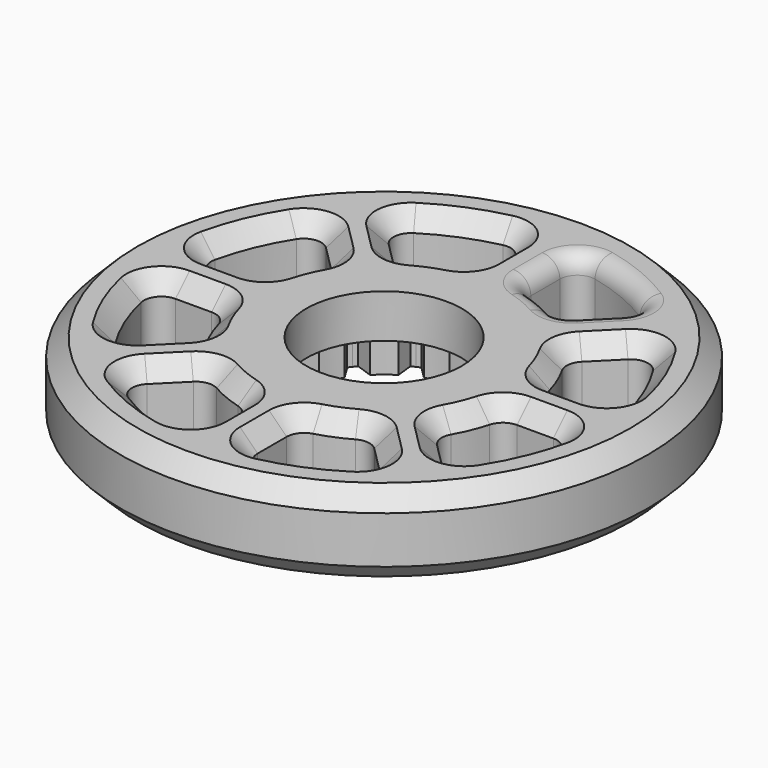
from build123d import *

# Parameters (mm, degrees)
F0_R     = 75
F0_R_2   = 22.1
F1_DEPTH = 23.4
F2_R     = 22.1
F3_DEPTH = 11
F5_DEPTH = 25
F6_F1_R  = 5
F6_F2_R  = 5
F7_SIZE  = 5


with BuildPart() as f1:
    # F0 (on Top) → F1 (new body)
    with BuildSketch(Plane.XY):
        Circle(F0_R)
        Circle(F0_R_2, mode=Mode.SUBTRACT)
    extrude(amount=F1_DEPTH)

    # F2 (on face) → F3 (cut)
    with BuildSketch(Plane(origin=(0, 0, 0), x_dir=(1, 0, 0), z_dir=(0, 0, -1))):
        with BuildLine():
            Line((1.25, -31.4751886412), (2.9, -26.8438074796))
            ThreePointArc((2.9, -26.8438074796), (6.0080652168, -26.3230536289), (9.0342818445, -25.4436976785))
            Line((9.0342818445, -25.4436976785), (12.5303614522, -28.900519751))
            Line((12.5303614522, -28.900519751), (13.6673377822, -28.3805193389))
            Line((13.6673377822, -28.3805193389), (14.782783622, -27.8158104032))
            Line((14.782783622, -27.8158104032), (14.2599012783, -22.9271719916))
            ThreePointArc((14.2599012783, -22.9271719916), (16.8342246502, -21.1094500266), (19.1792133714, -19.0041515057))
            Line((19.1792133714, -19.0041515057), (23.828931144, -20.6017484825))
            Line((23.828931144, -20.6017484825), (24.6276916977, -19.6399287586))
            Line((24.6276916977, -19.6399287586), (25.3876556486, -18.6471697763))
            Line((25.3876556486, -18.6471697763), (22.7954542222, -14.4695289074))
            ThreePointArc((22.7954542222, -14.4695289074), (24.3261594334, -11.7148609562), (25.5254664726, -8.8006000566))
            Line((25.5254664726, -8.8006000566), (30.4078887801, -8.2225482631))
            Line((30.4078887801, -8.2225482631), (30.7102292337, -7.0094094196))
            Line((30.7102292337, -7.0094094196), (30.964191115, -5.7852284827))
            Line((30.964191115, -5.7852284827), (26.8160878895, -3.146018166))
            ThreePointArc((26.8160878895, -3.146018166), (27, 0), (26.8160878895, 3.146018166))
            Line((26.8160878895, 3.146018166), (30.964191115, 5.7852284827))
            Line((30.964191115, 5.7852284827), (30.7102292337, 7.0094094196))
            Line((30.7102292337, 7.0094094196), (30.4078887801, 8.2225482631))
            Line((30.4078887801, 8.2225482631), (25.5254664726, 8.8006000566))
            ThreePointArc((25.5254664726, 8.8006000566), (24.3261594334, 11.7148609562), (22.7954542222, 14.4695289074))
            Line((22.7954542222, 14.4695289074), (25.3876556486, 18.6471697763))
            Line((25.3876556486, 18.6471697763), (24.6276916977, 19.6399287586))
            Line((24.6276916977, 19.6399287586), (23.828931144, 20.6017484825))
            Line((23.828931144, 20.6017484825), (19.1792133714, 19.0041515057))
            ThreePointArc((19.1792133714, 19.0041515057), (16.8342246502, 21.1094500266), (14.2599012783, 22.9271719916))
            Line((14.2599012783, 22.9271719916), (14.782783622, 27.8158104032))
            Line((14.782783622, 27.8158104032), (13.6673377822, 28.3805193389))
            Line((13.6673377822, 28.3805193389), (12.5303614522, 28.900519751))
            Line((12.5303614522, 28.900519751), (9.0342818445, 25.4436976785))
            ThreePointArc((9.0342818445, 25.4436976785), (6.0080652168, 26.3230536289), (2.9, 26.8438074796))
            Line((2.9, 26.8438074796), (1.25, 31.4751886412))
            Line((1.25, 31.4751886412), (0, 31.5))
            Line((0, 31.5), (-1.25, 31.4751886412))
            Line((-1.25, 31.4751886412), (-2.9, 26.8438074796))
            ThreePointArc((-2.9, 26.8438074796), (-6.0080652168, 26.3230536289), (-9.0342818445, 25.4436976785))
            Line((-9.0342818445, 25.4436976785), (-12.5303614522, 28.900519751))
            Line((-12.5303614522, 28.900519751), (-13.6673377822, 28.3805193389))
            Line((-13.6673377822, 28.3805193389), (-14.782783622, 27.8158104032))
            Line((-14.782783622, 27.8158104032), (-14.2599012783, 22.9271719916))
            ThreePointArc((-14.2599012783, 22.9271719916), (-16.8342246502, 21.1094500266), (-19.1792133714, 19.0041515057))
            Line((-19.1792133714, 19.0041515057), (-23.828931144, 20.6017484825))
            Line((-23.828931144, 20.6017484825), (-24.6276916977, 19.6399287586))
            Line((-24.6276916977, 19.6399287586), (-25.3876556486, 18.6471697763))
            Line((-25.3876556486, 18.6471697763), (-22.7954542222, 14.4695289074))
            ThreePointArc((-22.7954542222, 14.4695289074), (-24.3261594334, 11.7148609562), (-25.5254664726, 8.8006000566))
            Line((-25.5254664726, 8.8006000566), (-30.4078887801, 8.2225482631))
            Line((-30.4078887801, 8.2225482631), (-30.7102292337, 7.0094094196))
            Line((-30.7102292337, 7.0094094196), (-30.964191115, 5.7852284827))
            Line((-30.964191115, 5.7852284827), (-26.8160878895, 3.146018166))
            ThreePointArc((-26.8160878895, 3.146018166), (-27, 0), (-26.8160878895, -3.146018166))
            Line((-26.8160878895, -3.146018166), (-30.964191115, -5.7852284827))
            Line((-30.964191115, -5.7852284827), (-30.7102292337, -7.0094094196))
            Line((-30.7102292337, -7.0094094196), (-30.4078887801, -8.2225482631))
            Line((-30.4078887801, -8.2225482631), (-25.5254664726, -8.8006000566))
            ThreePointArc((-25.5254664726, -8.8006000566), (-24.3261594334, -11.7148609562), (-22.7954542222, -14.4695289074))
            Line((-22.7954542222, -14.4695289074), (-25.3876556486, -18.6471697763))
            Line((-25.3876556486, -18.6471697763), (-24.6276916977, -19.6399287586))
            Line((-24.6276916977, -19.6399287586), (-23.828931144, -20.6017484825))
            Line((-23.828931144, -20.6017484825), (-19.1792133714, -19.0041515057))
            ThreePointArc((-19.1792133714, -19.0041515057), (-16.8342246502, -21.1094500266), (-14.2599012783, -22.9271719916))
            Line((-14.2599012783, -22.9271719916), (-14.782783622, -27.8158104032))
            Line((-14.782783622, -27.8158104032), (-13.6673377822, -28.3805193389))
            Line((-13.6673377822, -28.3805193389), (-12.5303614522, -28.900519751))
            Line((-12.5303614522, -28.900519751), (-9.0342818445, -25.4436976785))
            ThreePointArc((-9.0342818445, -25.4436976785), (-6.0080652168, -26.3230536289), (-2.9, -26.8438074796))
            Line((-2.9, -26.8438074796), (-1.25, -31.4751886412))
            Line((-1.25, -31.4751886412), (0, -31.5))
            Line((0, -31.5), (1.25, -31.4751886412))
        make_face()
        Circle(F2_R, mode=Mode.SUBTRACT)
        with BuildLine():
            ThreePointArc((0, -31.5), (0.6251231086, -31.4937965495), (1.25, -31.4751886412))
            Line((1.25, -31.4751886412), (0, -31.5))
        make_face()
        with BuildLine():
            Line((13.6673377822, -28.3805193389), (12.5303614522, -28.900519751))
            ThreePointArc((12.5303614522, -28.900519751), (13.1014297465, -28.6461609749), (13.6673377822, -28.3805193389))
        make_face()
        with BuildLine():
            Line((14.782783622, -27.8158104032), (13.6673377822, -28.3805193389))
            ThreePointArc((13.6673377822, -28.3805193389), (14.2278626653, -28.1036994714), (14.782783622, -27.8158104032))
        make_face()
        with BuildLine():
            ThreePointArc((-13.6673377822, -28.3805193389), (-13.1014297465, -28.6461609749), (-12.5303614522, -28.900519751))
            Line((-12.5303614522, -28.900519751), (-13.6673377822, -28.3805193389))
        make_face()
        with BuildLine():
            Line((24.6276916977, -19.6399287586), (23.828931144, -20.6017484825))
            ThreePointArc((23.828931144, -20.6017484825), (24.2330837617, -20.1248018971), (24.6276916977, -19.6399287586))
        make_face()
        with BuildLine():
            ThreePointArc((-14.782783622, -27.8158104032), (-14.2278626653, -28.1036994714), (-13.6673377822, -28.3805193389))
            Line((-13.6673377822, -28.3805193389), (-14.782783622, -27.8158104032))
        make_face()
        with BuildLine():
            Line((25.3876556486, -18.6471697763), (24.6276916977, -19.6399287586))
            ThreePointArc((24.6276916977, -19.6399287586), (25.0125995279, -19.1473200437), (25.3876556486, -18.6471697763))
        make_face()
        with BuildLine():
            Line((30.7102292337, -7.0094094196), (30.4078887801, -8.2225482631))
            ThreePointArc((30.4078887801, -8.2225482631), (30.5650783387, -7.6174789891), (30.7102292337, -7.0094094196))
        make_face()
        with BuildLine():
            ThreePointArc((-25.3876556486, -18.6471697763), (-25.0125995279, -19.1473200437), (-24.6276916977, -19.6399287586))
            Line((-24.6276916977, -19.6399287586), (-25.3876556486, -18.6471697763))
        make_face()
        with BuildLine():
            Line((30.964191115, -5.7852284827), (30.7102292337, -7.0094094196))
            ThreePointArc((30.7102292337, -7.0094094196), (30.8432842946, -6.3985790549), (30.964191115, -5.7852284827))
        make_face()
        with BuildLine():
            Line((30.7102292337, 7.0094094196), (30.964191115, 5.7852284827))
            ThreePointArc((30.964191115, 5.7852284827), (30.8432842946, 6.3985790549), (30.7102292337, 7.0094094196))
        make_face()
        with BuildLine():
            ThreePointArc((-30.964191115, -5.7852284827), (-30.8432842946, -6.3985790549), (-30.7102292337, -7.0094094196))
            Line((-30.7102292337, -7.0094094196), (-30.964191115, -5.7852284827))
        make_face()
        with BuildLine():
            Line((30.4078887801, 8.2225482631), (30.7102292337, 7.0094094196))
            ThreePointArc((30.7102292337, 7.0094094196), (30.5650783387, 7.6174789891), (30.4078887801, 8.2225482631))
        make_face()
        with BuildLine():
            ThreePointArc((-30.7102292337, 7.0094094196), (-30.8432842946, 6.3985790549), (-30.964191115, 5.7852284827))
            Line((-30.964191115, 5.7852284827), (-30.7102292337, 7.0094094196))
        make_face()
        with BuildLine():
            Line((24.6276916977, 19.6399287586), (25.3876556486, 18.6471697763))
            ThreePointArc((25.3876556486, 18.6471697763), (25.0125995279, 19.1473200437), (24.6276916977, 19.6399287586))
        make_face()
        with BuildLine():
            ThreePointArc((-30.4078887801, 8.2225482631), (-30.5650783387, 7.6174789891), (-30.7102292337, 7.0094094196))
            Line((-30.7102292337, 7.0094094196), (-30.4078887801, 8.2225482631))
        make_face()
        with BuildLine():
            Line((23.828931144, 20.6017484825), (24.6276916977, 19.6399287586))
            ThreePointArc((24.6276916977, 19.6399287586), (24.2330837617, 20.1248018971), (23.828931144, 20.6017484825))
        make_face()
        with BuildLine():
            ThreePointArc((-24.6276916977, 19.6399287586), (-25.0125995279, 19.1473200437), (-25.3876556486, 18.6471697763))
            Line((-25.3876556486, 18.6471697763), (-24.6276916977, 19.6399287586))
        make_face()
        with BuildLine():
            Line((13.6673377822, 28.3805193389), (14.782783622, 27.8158104032))
            ThreePointArc((14.782783622, 27.8158104032), (14.2278626653, 28.1036994714), (13.6673377822, 28.3805193389))
        make_face()
        with BuildLine():
            ThreePointArc((-23.828931144, 20.6017484825), (-24.2330837617, 20.1248018971), (-24.6276916977, 19.6399287586))
            Line((-24.6276916977, 19.6399287586), (-23.828931144, 20.6017484825))
        make_face()
        with BuildLine():
            Line((12.5303614522, 28.900519751), (13.6673377822, 28.3805193389))
            ThreePointArc((13.6673377822, 28.3805193389), (13.1014297465, 28.6461609749), (12.5303614522, 28.900519751))
        make_face()
        with BuildLine():
            ThreePointArc((-13.6673377822, 28.3805193389), (-14.2278626653, 28.1036994714), (-14.782783622, 27.8158104032))
            Line((-14.782783622, 27.8158104032), (-13.6673377822, 28.3805193389))
        make_face()
        with BuildLine():
            Line((0, 31.5), (1.25, 31.4751886412))
            ThreePointArc((1.25, 31.4751886412), (0.6251231086, 31.4937965495), (0, 31.5))
        make_face()
        with BuildLine():
            ThreePointArc((-12.5303614522, 28.900519751), (-13.1014297465, 28.6461609749), (-13.6673377822, 28.3805193389))
            Line((-13.6673377822, 28.3805193389), (-12.5303614522, 28.900519751))
        make_face()
        with BuildLine():
            Line((-1.25, 31.4751886412), (0, 31.5))
            ThreePointArc((0, 31.5), (-0.6251231086, 31.4937965495), (-1.25, 31.4751886412))
        make_face()
    extrude(amount=-F3_DEPTH, mode=Mode.SUBTRACT)

    # F4 (on face) → F5 (cut)
    with BuildSketch(Plane(origin=(0, 0, 0), x_dir=(1, 0, 0), z_dir=(0, 0, -1))):
        with BuildLine():
            ThreePointArc((-39.3817561055, 7.0055182569), (-36.9551813005, 15.3073372946), (-32.8007562624, 22.893457332))
            Line((-32.8007562624, 22.893457332), (-47.0898732753, 37.1825743449))
            ThreePointArc((-47.0898732753, 37.1825743449), (-55.4327719507, 22.9610059419), (-59.5896191795, 7.0055182569))
            Line((-59.5896191795, 7.0055182569), (-39.3817561055, 7.0055182569))
        make_face()
        with BuildLine():
            Line((-7.0055182569, 39.3817561055), (-7.0055182569, 59.5896191795))
            ThreePointArc((-7.0055182569, 59.5896191795), (-22.9610059419, 55.4327719507), (-37.1825743449, 47.0898732753))
            Line((-37.1825743449, 47.0898732753), (-22.893457332, 32.8007562624))
            ThreePointArc((-22.893457332, 32.8007562624), (-15.3073372946, 36.9551813005), (-7.0055182569, 39.3817561055))
        make_face()
        with BuildLine():
            ThreePointArc((37.1825743449, 47.0898732753), (22.9610059419, 55.4327719507), (7.0055182569, 59.5896191795))
            Line((7.0055182569, 59.5896191795), (7.0055182569, 39.3817561055))
            ThreePointArc((7.0055182569, 39.3817561055), (15.3073372946, 36.9551813005), (22.893457332, 32.8007562624))
            Line((22.893457332, 32.8007562624), (37.1825743449, 47.0898732753))
        make_face()
        with BuildLine():
            Line((39.3817561055, 7.0055182569), (59.5896191795, 7.0055182569))
            ThreePointArc((59.5896191795, 7.0055182569), (55.4327719507, 22.9610059419), (47.0898732753, 37.1825743449))
            Line((47.0898732753, 37.1825743449), (32.8007562624, 22.893457332))
            ThreePointArc((32.8007562624, 22.893457332), (36.9551813005, 15.3073372946), (39.3817561055, 7.0055182569))
        make_face()
        with BuildLine():
            Line((32.8007562624, -22.893457332), (47.0898732753, -37.1825743449))
            ThreePointArc((47.0898732753, -37.1825743449), (55.4327719507, -22.9610059419), (59.5896191795, -7.0055182569))
            Line((59.5896191795, -7.0055182569), (39.3817561055, -7.0055182569))
            ThreePointArc((39.3817561055, -7.0055182569), (36.9551813005, -15.3073372946), (32.8007562624, -22.893457332))
        make_face()
        with BuildLine():
            Line((7.0055182569, -39.3817561055), (7.0055182569, -59.5896191795))
            ThreePointArc((7.0055182569, -59.5896191795), (22.9610059419, -55.4327719507), (37.1825743449, -47.0898732753))
            Line((37.1825743449, -47.0898732753), (22.893457332, -32.8007562624))
            ThreePointArc((22.893457332, -32.8007562624), (15.3073372946, -36.9551813005), (7.0055182569, -39.3817561055))
        make_face()
        with BuildLine():
            Line((-22.893457332, -32.8007562624), (-37.1825743449, -47.0898732753))
            ThreePointArc((-37.1825743449, -47.0898732753), (-22.9610059419, -55.4327719507), (-7.0055182569, -59.5896191795))
            Line((-7.0055182569, -59.5896191795), (-7.0055182569, -39.3817561055))
            ThreePointArc((-7.0055182569, -39.3817561055), (-15.3073372946, -36.9551813005), (-22.893457332, -32.8007562624))
        make_face()
        with BuildLine():
            Line((-39.3817561055, -7.0055182569), (-59.5896191795, -7.0055182569))
            ThreePointArc((-59.5896191795, -7.0055182569), (-55.4327719507, -22.9610059419), (-47.0898732753, -37.1825743449))
            Line((-47.0898732753, -37.1825743449), (-32.8007562624, -22.893457332))
            ThreePointArc((-32.8007562624, -22.893457332), (-36.9551813005, -15.3073372946), (-39.3817561055, -7.0055182569))
        make_face()
    extrude(amount=-F5_DEPTH, mode=Mode.SUBTRACT)

    # F6: fillet of radius 5 on 34 edges, made by hand

    # F6_f1
    f6_f1_edges = [f1.edges().sort_by_distance(p)[0] for p in [
        (-47.0898732753, -37.1825743449, 11.7),
        (-37.1825743449, -47.0898732753, 11.7),
        (-32.8007562624, -22.893457332, 11.7),
        (-7.0055182569, -39.3817561055, 11.7),
        (-39.3817561055, -7.0055182569, 11.7),
        (22.893457332, -32.8007562624, 11.7),
        (37.1825743449, 47.0898732753, 11.7),
        (-32.8007562624, 22.893457332, 11.7),
        (-7.0055182569, 39.3817561055, 11.7),
        (-39.3817561055, 7.0055182569, 11.7),
        (-22.893457332, 32.8007562624, 11.7),
        (7.0055182569, 39.3817561055, 11.7),
        (22.893457332, 32.8007562624, 11.7),
        (32.8007562624, 22.893457332, 11.7),
        (39.3817561055, 7.0055182569, 11.7),
        (39.3817561055, -7.0055182569, 11.7),
        (32.8007562624, -22.893457332, 11.7),
        (7.0055182569, -39.3817561055, 11.7),
        (-22.893457332, -32.8007562624, 11.7),
        (47.0898732753, 37.1825743449, 11.7),
        (7.0055182569, 59.5896191795, 11.7),
        (-7.0055182569, 59.5896191795, 11.7),
        (-37.1825743449, 47.0898732753, 11.7),
        (-47.0898732753, 37.1825743449, 11.7),
        (-59.5896191795, 7.0055182569, 11.7),
        (-59.5896191795, -7.0055182569, 11.7),
        (-7.0055182569, -59.5896191795, 11.7),
        (7.0055182569, -59.5896191795, 11.7),
        (37.1825743449, -47.0898732753, 11.7),
        (47.0898732753, -37.1825743449, 11.7),
        (59.5896191795, -7.0055182569, 11.7),
        (59.5896191795, 7.0055182569, 11.7),
    ]]
    fillet(f6_f1_edges, radius=F6_F1_R)

    # F6_f2
    f6_f2_edges = [f1.edges().sort_by_distance(p)[0] for p in [
        (22.9610059419, 55.4327719507, 0),
        (22.9610059419, 55.4327719507, 23.4),
        (8.8795826972, 57.5760881156, 23.4),
        (34.4336292014, 46.99125548, 23.4),
        (8.8795826972, 57.5760881156, 0),
        (34.4336292014, 46.99125548, 0),
    ]]
    fillet(f6_f2_edges, radius=F6_F2_R)

    # F7
    f7_edges = [f1.edges().sort_by_distance(p)[0] for p in [
        (-75, 0, 23.4),
        (-75, 0, 0),
        (-22.961006, 55.432772, 0),
        (-55.432772, 22.961006, 0),
        (-58.553142, 13.096929, 11.7),
        (-50.664251, 32.142397, 11.7),
        (-55.432772, 22.961006, 23.4),
        (-32.142397, 50.664251, 11.7),
        (-13.096929, 58.553142, 11.7),
        (-22.961006, 55.432772, 23.4),
        (-55.432772, -22.961006, 0),
        (-50.664251, -32.142397, 11.7),
        (-58.553142, -13.096929, 11.7),
        (-55.432772, -22.961006, 23.4),
        (-22.961006, -55.432772, 0),
        (-13.096929, -58.553142, 11.7),
        (-32.142397, -50.664251, 11.7),
        (-22.961006, -55.432772, 23.4),
        (22.961006, -55.432772, 0),
        (32.142397, -50.664251, 11.7),
        (13.096929, -58.553142, 11.7),
        (22.961006, -55.432772, 23.4),
        (39.263419, -29.35612, 0),
        (42.906696, -32.999397, 11.7),
        (35.620142, -25.712843, 11.7),
        (39.263419, -29.35612, 23.4),
        (39.263419, 29.35612, 23.4),
        (39.263419, 29.35612, 0),
        (35.620142, 25.712843, 11.7),
        (42.906696, 32.999397, 11.7),
    ]]
    chamfer(f7_edges, length=F7_SIZE)


solid = f1.part
